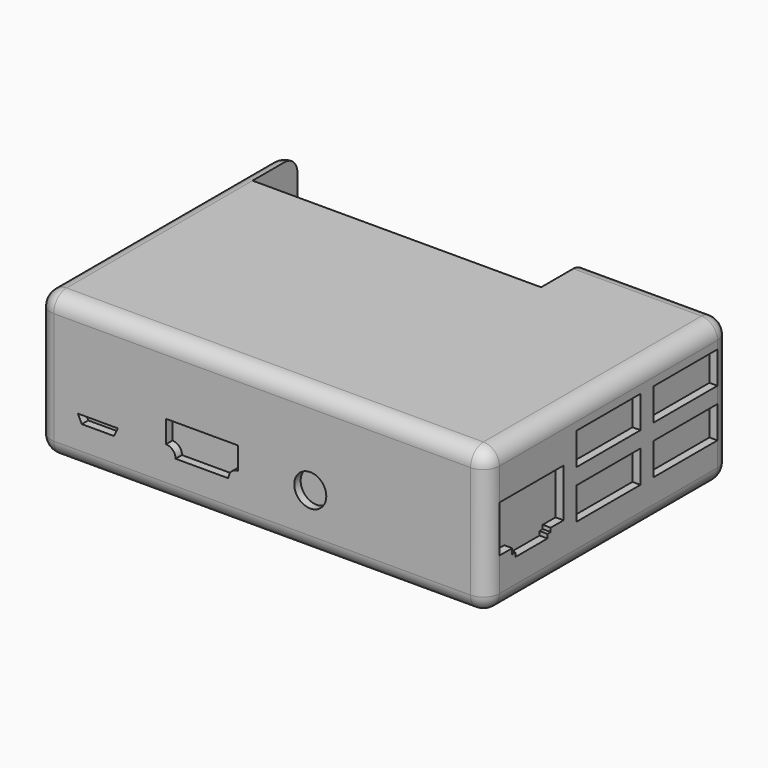
from build123d import *

# Parameters (mm, degrees)
F0_W     = 6.35
F0_H     = 7.14375
F1_DEPTH = 28.575
F2_DEPTH = 6.35
F4_W     = 15.875
F4_H     = 6.35
F5_DEPTH = 1.5875
F3_R     = 3.175
F6_DEPTH = 1.5875
F7_W     = 57.15
F7_H     = 11.1125
F8_DEPTH = 11.1125
F9_R     = 3.17499


# Not quite as in the source:
# - a fillet or chamfer is up to 0.001 mm smaller than in the source, because OpenCascade refuses the exact size


with BuildPart() as f1:
    # F0 (on Top) → F1 (new body)
    with BuildSketch(Plane.XY):
        Polygon((44.45, -30.1625), (44.45, 30.1625), (-44.45, 30.1625), (-44.45, 7.14375), (-38.1, 7.14375), (-38.1, 0), (-38.1, -7.14375), (-44.45, -7.14375), (-44.45, -30.1625), align=None)
        with BuildLine():
            add(Edge.make_bspline(
                [(-14.2875, 0), (-14.2875, 0.7324493897), (-15.9479784808, 2.0808128457), (-17.5976715514, 0.8021829538), (-21.43125, 5.9657530394), (-25.2648284486, 0.8021829538), (-26.9145215192, 2.0808128457), (-29.4769945213, 0), (-26.9145215192, -2.0808128457), (-25.2648284486, -0.8021829538), (-21.43125, -5.9657530394), (-17.5976715514, -0.8021829538), (-15.9479784808, -2.0808128457), (-14.2875, -0.7324493897), (-14.2875, 0)],
                knots=[0, 0, 0, 0, 0.0762961044, 0.1404532251, 0.25, 0.3595467749, 0.4237038956, 0.5, 0.5762961044, 0.6404532251, 0.75, 0.8595467749, 0.9237038956, 1, 1, 1, 1], degree=3))
        make_face(mode=Mode.SUBTRACT)
        with BuildLine():
            add(Edge.make_bspline(
                [(14.2875, 0), (14.2875, 0.7324493897), (15.9479784808, 2.0808128457), (17.5976715514, 0.8021829538), (21.43125, 5.9657530394), (25.2648284486, 0.8021829538), (26.9145215192, 2.0808128457), (29.4769945213, 0), (26.9145215192, -2.0808128457), (25.2648284486, -0.8021829538), (21.43125, -5.9657530394), (17.5976715514, -0.8021829538), (15.9479784808, -2.0808128457), (14.2875, -0.7324493897), (14.2875, 0)],
                knots=[0, 0, 0, 0, 0.0762961044, 0.1404532251, 0.25, 0.3595467749, 0.4237038956, 0.5, 0.5762961044, 0.6404532251, 0.75, 0.8595467749, 0.9237038956, 1, 1, 1, 1], degree=3))
        make_face(mode=Mode.SUBTRACT)
        with Locations((-41.275, 3.571875)):
            Rectangle(F0_W, F0_H)
        with Locations((-41.275, -3.571875)):
            Rectangle(F0_W, F0_H)
        with BuildLine():
            add(Edge.make_bspline(
                [(-14.2875, 0), (-14.2875, 0.7324493897), (-15.9479784808, 2.0808128457), (-17.5976715514, 0.8021829538), (-21.43125, 5.9657530394), (-25.2648284486, 0.8021829538), (-26.9145215192, 2.0808128457), (-29.4769945213, 0), (-26.9145215192, -2.0808128457), (-25.2648284486, -0.8021829538), (-21.43125, -5.9657530394), (-17.5976715514, -0.8021829538), (-15.9479784808, -2.0808128457), (-14.2875, -0.7324493897), (-14.2875, 0)],
                knots=[0, 0, 0, 0, 0.0762961044, 0.1404532251, 0.25, 0.3595467749, 0.4237038956, 0.5, 0.5762961044, 0.6404532251, 0.75, 0.8595467749, 0.9237038956, 1, 1, 1, 1], degree=3))
        make_face()
        with BuildLine():
            add(Edge.make_bspline(
                [(14.2875, 0), (14.2875, 0.7324493897), (15.9479784808, 2.0808128457), (17.5976715514, 0.8021829538), (21.43125, 5.9657530394), (25.2648284486, 0.8021829538), (26.9145215192, 2.0808128457), (29.4769945213, 0), (26.9145215192, -2.0808128457), (25.2648284486, -0.8021829538), (21.43125, -5.9657530394), (17.5976715514, -0.8021829538), (15.9479784808, -2.0808128457), (14.2875, -0.7324493897), (14.2875, 0)],
                knots=[0, 0, 0, 0, 0.0762961044, 0.1404532251, 0.25, 0.3595467749, 0.4237038956, 0.5, 0.5762961044, 0.6404532251, 0.75, 0.8595467749, 0.9237038956, 1, 1, 1, 1], degree=3))
        make_face()
    extrude(amount=F1_DEPTH)

    # F0 (on Top) → F2 (cut)
    with BuildSketch(Plane.XY):
        with Locations((-41.275, 3.571875)):
            Rectangle(F0_W, F0_H)
        with Locations((-41.275, -3.571875)):
            Rectangle(F0_W, F0_H)
        with BuildLine():
            add(Edge.make_bspline(
                [(-14.2875, 0), (-14.2875, 0.7324493897), (-15.9479784808, 2.0808128457), (-17.5976715514, 0.8021829538), (-21.43125, 5.9657530394), (-25.2648284486, 0.8021829538), (-26.9145215192, 2.0808128457), (-29.4769945213, 0), (-26.9145215192, -2.0808128457), (-25.2648284486, -0.8021829538), (-21.43125, -5.9657530394), (-17.5976715514, -0.8021829538), (-15.9479784808, -2.0808128457), (-14.2875, -0.7324493897), (-14.2875, 0)],
                knots=[0, 0, 0, 0, 0.0762961044, 0.1404532251, 0.25, 0.3595467749, 0.4237038956, 0.5, 0.5762961044, 0.6404532251, 0.75, 0.8595467749, 0.9237038956, 1, 1, 1, 1], degree=3))
        make_face()
        with BuildLine():
            add(Edge.make_bspline(
                [(14.2875, 0), (14.2875, 0.7324493897), (15.9479784808, 2.0808128457), (17.5976715514, 0.8021829538), (21.43125, 5.9657530394), (25.2648284486, 0.8021829538), (26.9145215192, 2.0808128457), (29.4769945213, 0), (26.9145215192, -2.0808128457), (25.2648284486, -0.8021829538), (21.43125, -5.9657530394), (17.5976715514, -0.8021829538), (15.9479784808, -2.0808128457), (14.2875, -0.7324493897), (14.2875, 0)],
                knots=[0, 0, 0, 0, 0.0762961044, 0.1404532251, 0.25, 0.3595467749, 0.4237038956, 0.5, 0.5762961044, 0.6404532251, 0.75, 0.8595467749, 0.9237038956, 1, 1, 1, 1], degree=3))
        make_face()
    extrude(amount=F2_DEPTH, mode=Mode.SUBTRACT)

    # F4 (on face) → F5 (cut)
    with BuildSketch(Plane.YZ.offset(44.45)):
        with Locations((19.05, 11.1125)):
            Rectangle(F4_W, F4_H)
        with Locations((19.05, 20.6375)):
            Rectangle(F4_W, F4_H)
        with Locations((0, 11.1125)):
            Rectangle(F4_W, F4_H)
        with Locations((0, 20.6375)):
            Rectangle(F4_W, F4_H)
        Polygon((-11.1125, 19.05), (-26.9875, 19.05), (-26.9875, 9.7991283983), (-23.8125, 9.7991283983), (-23.8125, 8.73125), (-23.01875, 8.73125), (-23.01875, 7.9375), (-15.08125, 7.9375), (-15.08125, 8.73125), (-14.2875, 8.73125), (-14.2875, 9.4989752397), (-11.1125, 9.4989752397), align=None)
    extrude(amount=-F5_DEPTH, mode=Mode.SUBTRACT)

    # F3 (on face) → F6 (cut)
    with BuildSketch(Plane.XZ.offset(30.1625)):
        Polygon((-28.575, 9.525), (-36.5125, 9.525), (-35.71875, 7.9375), (-29.36875, 7.9375), align=None)
        with BuildLine():
            Line((-4.7625, 14.2875), (-19.05, 14.2875))
            Line((-19.05, 14.2875), (-19.05, 9.8425))
            ThreePointArc((-19.05, 9.8425), (-17.7029615818, 9.2845384182), (-17.145, 7.9375))
            Line((-17.145, 7.9375), (-6.6675, 7.9375))
            ThreePointArc((-6.6675, 7.9375), (-6.1095384182, 9.2845384182), (-4.7625, 9.8425))
            Line((-4.7625, 9.8425), (-4.7625, 14.2875))
        make_face()
        with Locations((9.525, 11.1125)):
            Circle(F3_R)
    extrude(amount=-F6_DEPTH, mode=Mode.SUBTRACT)

    # F7 (on face) → F8 (cut)
    with BuildSketch(Plane.XY.offset(28.575)):
        with Locations((-12.7, 24.60625)):
            Rectangle(F7_W, F7_H)
    extrude(amount=-F8_DEPTH, mode=Mode.SUBTRACT)

    # F9 (radius 3.175 in the source; OpenCascade refuses exactly that, so slightly less here)
    f9_edges = [f1.edges().sort_by_distance(p)[0] for p in [
        (0, -30.1625, 28.575),
        (-44.45, 0, 28.575),
        (44.45, 0, 28.575),
        (44.45, -30.1625, 14.2875),
        (0, -30.1625, 0),
        (44.45, 0, 0),
        (44.45, 30.1625, 14.2875),
        (-42.8625, 30.1625, 28.575),
        (30.1625, 30.1625, 28.575),
        (0, 30.1625, 0),
        (-44.45, 30.1625, 14.2875),
        (-44.45, 18.653125, 0),
        (-44.45, -18.653125, 0),
        (-44.45, -30.1625, 14.2875),
    ]]
    fillet(f9_edges, radius=F9_R)


solid = f1.part
